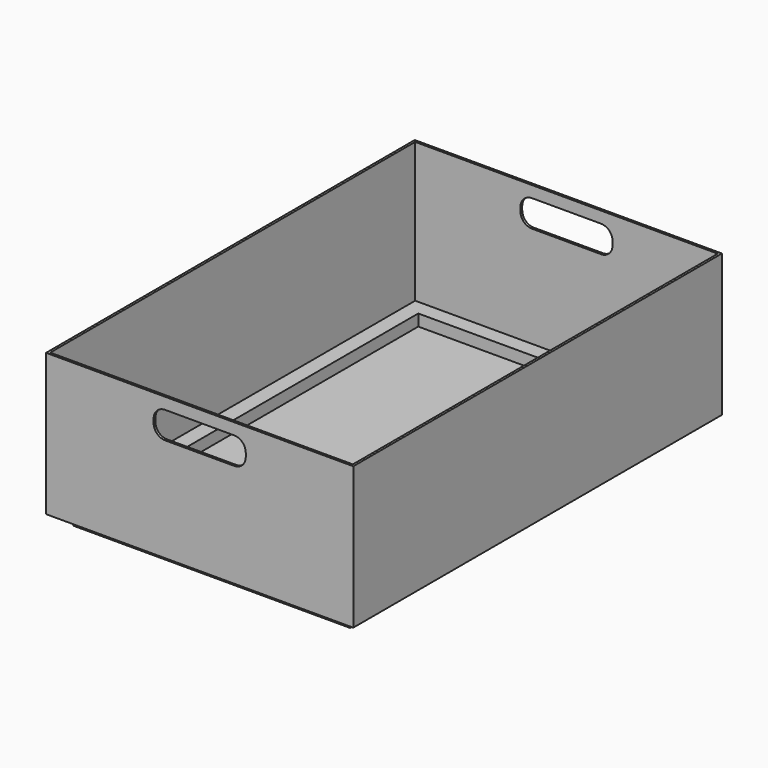
from build123d import *

# Parameters (mm, degrees)
F0_W     = 400
F0_H     = 200
F1_DEPTH = 300
F2_W     = 34.6541681295
F2_H     = 41.7717497936
F3_DEPTH = 600.001
F4_W     = 32.9372721782
F4_H     = 23.155899561
F5_DEPTH = 400.001
F6_T     = -3
F8_DEPTH = 600.001


# Not quite as in the source:
# - a pattern or mirror of a feature is missing from the dataset's text; its kind, count and spacing are read off the source's solid


with BuildPart() as f1:
    # F0 (on Front) → F1 (new body, symmetric)
    with BuildSketch(Plane.XZ):
        with Locations((0, 100)):
            Rectangle(F0_W, F0_H)
    extrude(amount=F1_DEPTH, both=True)

    # F2 (on face) → F3 (cut, through all)
    with BuildSketch(Plane.XZ.offset(300)):
        with Locations((-197.3270840647, -5.8858748968)):
            Rectangle(F2_W, F2_H)
    f3 = extrude(amount=-F3_DEPTH, mode=Mode.SUBTRACT)

    # F3_copies: F3 across plane
    add(f3.mirror(Plane(origin=(0, 0, 0), x_dir=(0, 0, 1), z_dir=(1, 0, 0))), mode=Mode.SUBTRACT)

    # F4 (on face) → F5 (cut, through all)
    with BuildSketch(Plane.YZ.offset(200)):
        with Locations((-296.4686360891, 3.4220502195)):
            Rectangle(F4_W, F4_H)
        with Locations((296.4686360891, 3.4220502195)):
            Rectangle(F4_W, F4_H)
    extrude(amount=-F5_DEPTH, mode=Mode.SUBTRACT)

    # F6
    f6_openings = [f1.faces().sort_by_distance(p)[0] for p in [
        (0, 0, 200),
    ]]
    offset(amount=F6_T, openings=f6_openings, kind=Kind.INTERSECTION)

    # F7 (on face) → F8 (cut, through all)
    with BuildSketch(Plane.XZ.offset(300)):
        with BuildLine():
            Line((45, 185), (-45, 185))
            ThreePointArc((-45, 185), (-55.6066017178, 180.6066017178), (-60, 170))
            Line((-60, 170), (-60, 165))
            ThreePointArc((-60, 165), (-55.6066017178, 154.3933982822), (-45, 150))
            Line((-45, 150), (45, 150))
            ThreePointArc((45, 150), (55.6066017178, 154.3933982822), (60, 165))
            Line((60, 165), (60, 170))
            ThreePointArc((60, 170), (55.6066017178, 180.6066017178), (45, 185))
        make_face()
    extrude(amount=-F8_DEPTH, mode=Mode.SUBTRACT)


solid = f1.part
